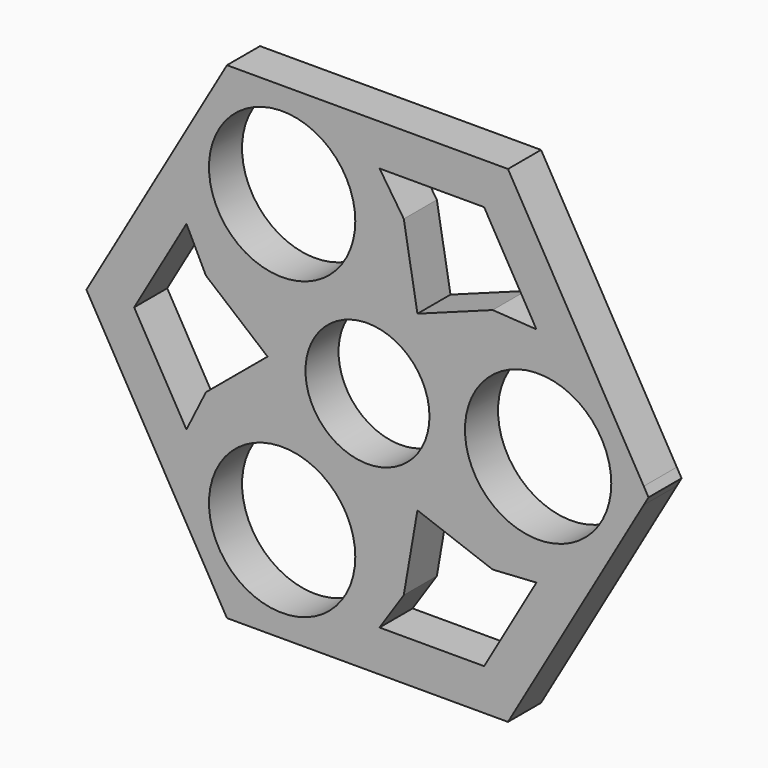
from build123d import *

# Parameters (mm, degrees)
F0_R     = 11.2395
F0_R_2   = 9.525
F1_DEPTH = 6.35


# Not quite as in the source:
# - ends of sketch curves that miss each other by under 0.0002 mm in the source are joined


with BuildPart() as f1:
    # F0 (on Front) → F1 (new body)
    with BuildSketch(Plane.XZ):
        with BuildLine():
            Line((42.4467651581, 1.27), (33.5675281941, 16.6492895541))
            Line((33.5675281941, 16.6492895541), (21.59, 37.3949769354))
            Line((21.59, 37.3949769354), (-2.3645964913, 37.3949769354))
            Line((-2.3645964913, 37.3949769354), (-20.1235303163, 37.3949769354))
            ThreePointArc((-20.1235303163, 37.3949769354), (-21.3935303163, 37.054681461), (-22.3232348419, 36.1249769354))
            Line((-22.3232348419, 36.1249769354), (-31.2024718059, 20.7456873813))
            Line((-31.2024718059, 20.7456873813), (-43.18, 0))
            Line((-43.18, 0), (-31.2027017544, -20.7452890988))
            Line((-31.2027017544, -20.7452890988), (-22.3232348418, -36.1249769356))
            ThreePointArc((-22.3232348418, -36.1249769356), (-21.9195815404, -36.6510281597), (-21.3935303163, -37.0546814611))
            ThreePointArc((-21.3935303163, -37.0546814611), (-20.7809306909, -37.3084285342), (-20.1235303165, -37.3949769354))
            Line((-20.1235303165, -37.3949769354), (-2.3645964913, -37.3949769354))
            Line((-2.3645964913, -37.3949769354), (21.59, -37.3949769354))
            Line((21.59, -37.3949769354), (33.5675281941, -16.6492895541))
            Line((33.5675281941, -16.6492895541), (42.4467651581, -1.27))
            ThreePointArc((42.4467651581, -1.27), (42.7870606325, 0), (42.4467651581, 1.27))
        make_face()
        with Locations((-13.1097560234, -22.7067635073)):
            Circle(F0_R, mode=Mode.SUBTRACT)
        Polygon((1.8552556307, -31.0449769354), (5.579663063, -25.4405181745), (7.6765207659, -13.2964418818), (19.2425445444, -17.5521669359), (25.957862804, -17.1289127727), (17.9235712565, -31.0449769354), align=None, mode=Mode.SUBTRACT)
        Polygon((-15.3532430276, -9.74608e-05), (-24.8219665561, -7.8881291301), (-24.8578663434, -7.9604670809), (-27.8131295737, -13.9154964701), (-35.8475243142, 0.000220433), (-27.8133665013, 13.915789961), (-24.8219665561, 7.8881291301), align=None, mode=Mode.SUBTRACT)
        with Locations((-13.1097560234, 22.7067635073)):
            Circle(F0_R, mode=Mode.SUBTRACT)
        Circle(F0_R_2, mode=Mode.SUBTRACT)
        with Locations((26.2195120463, 0.0001612286)):
            Circle(F0_R, mode=Mode.SUBTRACT)
        Polygon((7.6765207659, 13.2964418818), (5.579663063, 25.4405181745), (1.8552556307, 31.0449769354), (17.9235712565, 31.0449769354), (25.957862804, 17.1289127727), (19.2425445444, 17.5521669359), align=None, mode=Mode.SUBTRACT)
        with BuildLine():
            Line((43.18, 0), (42.4467651581, 1.27))
            ThreePointArc((42.4467651581, 1.27), (42.7870606325, 0), (42.4467651581, -1.27))
            Line((42.4467651581, -1.27), (43.18, 0))
        make_face()
        with BuildLine():
            ThreePointArc((-22.3232348419, 36.1249769354), (-21.3935303163, 37.054681461), (-20.1235303163, 37.3949769354))
            Line((-20.1235303163, 37.3949769354), (-21.59, 37.3949769354))
            Line((-21.59, 37.3949769354), (-22.3232348419, 36.1249769354))
        make_face()
        with BuildLine():
            Line((-21.59, -37.3949769354), (-20.1235303165, -37.3949769354))
            ThreePointArc((-20.1235303165, -37.3949769354), (-20.7809306909, -37.3084285342), (-21.3935303163, -37.0546814611))
            Line((-21.3935303163, -37.0546814611), (-21.59, -37.3949769354))
        make_face()
        with BuildLine():
            Line((-21.59, -37.3949769354), (-21.3935303163, -37.0546814611))
            ThreePointArc((-21.3935303163, -37.0546814611), (-21.9195815404, -36.6510281597), (-22.3232348418, -36.1249769356))
            Line((-22.3232348418, -36.1249769356), (-21.59, -37.3949769354))
        make_face()
    extrude(amount=F1_DEPTH)


solid = f1.part
